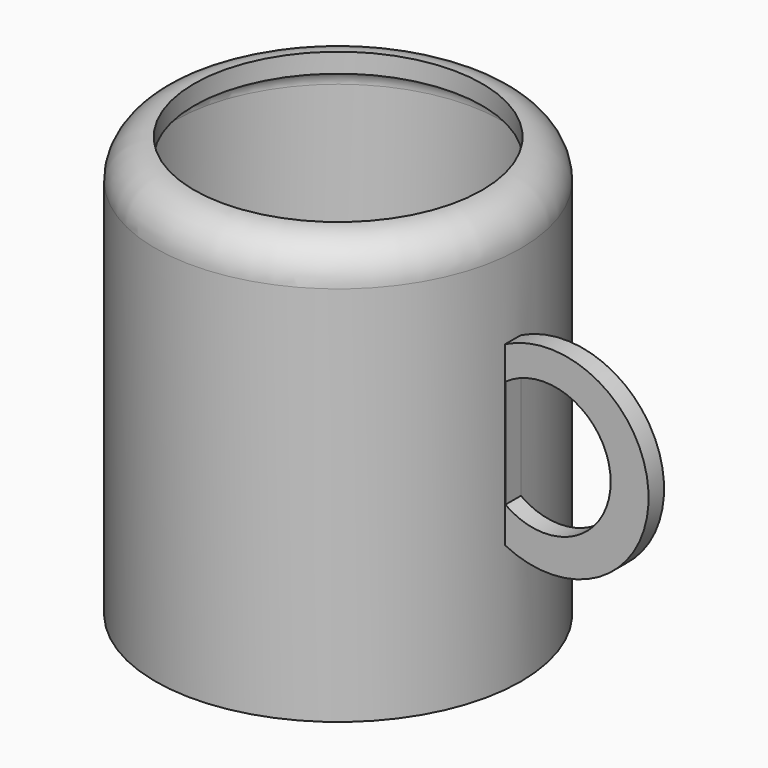
from build123d import *

# Parameters (mm, degrees)
F0_R     = 23.9903837703
F1_DEPTH = 55.118
F2_R     = 5.08
F3_T     = -2.54
F5_DEPTH = 2.54
F7_DEPTH = 4.1402


# Not quite as in the source:
# - a shell that OpenCascade refuses in one call is made with other operations: the cavity is built on its own and cut out


with BuildPart() as f1:
    # F0 (on Top) → F1 (new body)
    with BuildSketch(Plane.XY):
        Circle(F0_R)
    extrude(amount=F1_DEPTH)

    # F2
    f2_edges = [f1.edges().sort_by_distance(p)[0] for p in [
        (-23.990384, 0, 55.118),
    ]]
    fillet(f2_edges, radius=F2_R)

    # F3: a shell. OpenCascade refuses it in one call, so the cavity is built on its own and cut out:
    # the body offset inwards by the wall thickness, plus a prism from it out through each open face.
    f3_core = offset(f1.part, amount=F3_T, mode=Mode.PRIVATE)
    f3_exits = [f3_core.faces().sort_by_distance(p)[0] for p in [
        (0, 0, 52.578),
    ]]
    add(f3_core, mode=Mode.SUBTRACT)
    extrude(f3_exits, amount=-F3_T, mode=Mode.SUBTRACT)

    # F4 (on Front) → F5 (join)
    with BuildSketch(Plane.XZ):
        with BuildLine():
            ThreePointArc((23.9537265152, 16.7385414243), (42.7735621339, 28.3666290343), (23.9537265152, 39.9947166443))
            Line((23.9537265152, 39.9947166443), (23.9537265152, 16.7385414243))
        make_face()
    extrude(amount=F5_DEPTH)

    # F6 (on Front) → F7 (cut)
    with BuildSketch(Plane.XZ):
        with BuildLine():
            ThreePointArc((23.9792838693, 21.4542429894), (37.798657028, 28.5622673109), (23.9792838693, 35.6702916324))
            Line((23.9792838693, 35.6702916324), (23.9792838693, 21.4542429894))
        make_face()
    extrude(amount=F7_DEPTH, mode=Mode.SUBTRACT)


solid = f1.part
